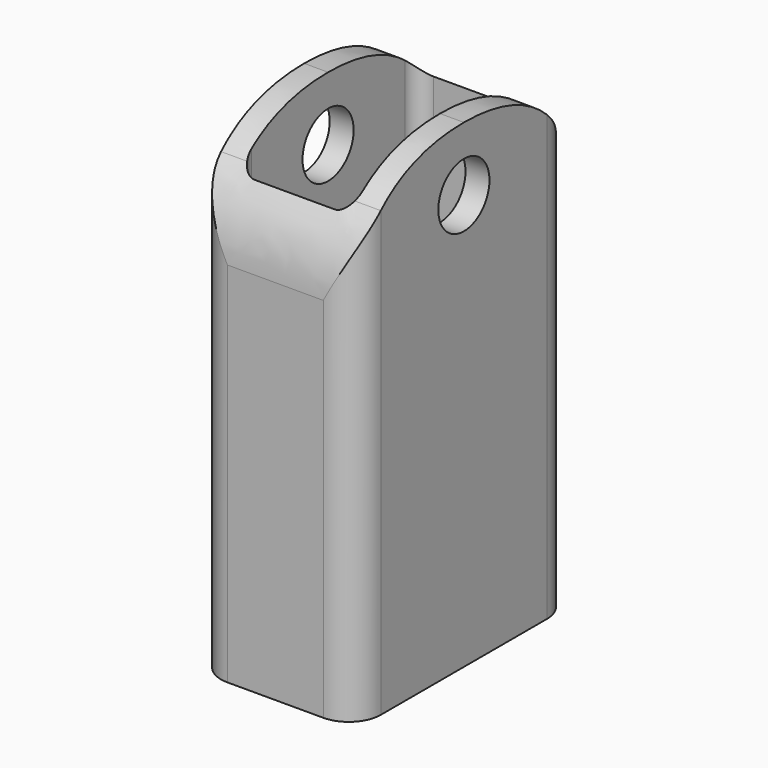
from build123d import *

# Parameters (mm, degrees)
F1_DEPTH     = 1.4
F2_DEPTH     = 30
F3_R         = 2
F4_DEPTH     = 10.001
F5_T4_DEPTH  = 22
F5_T10_DEPTH = 22


# Not quite as in the source:
# - a fillet or chamfer that OpenCascade refuses, or shapes differently, is made with other operations: its cross-section is extruded or revolved along the edge and cut away or added


with BuildPart() as f1:
    # F0 (on Top) → F1 (new body)
    with BuildSketch(Plane.XY):
        with BuildLine():
            ThreePointArc((5, 6.5), (4.4142135624, 7.9142135624), (3, 8.5))
            Line((3, 8.5), (-3, 8.5))
            ThreePointArc((-3, 8.5), (-4.4142135624, 7.9142135624), (-5, 6.5))
            Line((-5, 6.5), (-5, -6.5))
            ThreePointArc((-5, -6.5), (-4.4142135624, -7.9142135624), (-3, -8.5))
            Line((-3, -8.5), (3, -8.5))
            ThreePointArc((3, -8.5), (4.4142135624, -7.9142135624), (5, -6.5))
            Line((5, -6.5), (5, 6.5))
        make_face()
        with BuildLine():
            Line((-2.5, 7), (2.5, 7))
            ThreePointArc((2.5, 7), (3.2071067812, 6.7071067812), (3.5, 6))
            Line((3.5, 6), (3.5, -6))
            ThreePointArc((3.5, -6), (3.2071067812, -6.7071067812), (2.5, -7))
            Line((2.5, -7), (-2.5, -7))
            ThreePointArc((-2.5, -7), (-3.2071067812, -6.7071067812), (-3.5, -6))
            Line((-3.5, -6), (-3.5, 6))
            ThreePointArc((-3.5, 6), (-3.2071067812, 6.7071067812), (-2.5, 7))
        make_face(mode=Mode.SUBTRACT)
        with BuildLine():
            ThreePointArc((3.5, 6), (3.2071067812, 6.7071067812), (2.5, 7))
            Line((2.5, 7), (-2.5, 7))
            ThreePointArc((-2.5, 7), (-3.2071067812, 6.7071067812), (-3.5, 6))
            Line((-3.5, 6), (-3.5, -6))
            ThreePointArc((-3.5, -6), (-3.2071067812, -6.7071067812), (-2.5, -7))
            Line((-2.5, -7), (2.5, -7))
            ThreePointArc((2.5, -7), (3.2071067812, -6.7071067812), (3.5, -6))
            Line((3.5, -6), (3.5, 6))
        make_face()
    extrude(amount=F1_DEPTH)

    # F0 (on Top) → F2 (join)
    with BuildSketch(Plane.XY):
        with BuildLine():
            ThreePointArc((5, 6.5), (4.4142135624, 7.9142135624), (3, 8.5))
            Line((3, 8.5), (-3, 8.5))
            ThreePointArc((-3, 8.5), (-4.4142135624, 7.9142135624), (-5, 6.5))
            Line((-5, 6.5), (-5, -6.5))
            ThreePointArc((-5, -6.5), (-4.4142135624, -7.9142135624), (-3, -8.5))
            Line((-3, -8.5), (3, -8.5))
            ThreePointArc((3, -8.5), (4.4142135624, -7.9142135624), (5, -6.5))
            Line((5, -6.5), (5, 6.5))
        make_face()
        with BuildLine():
            Line((-2.5, 7), (2.5, 7))
            ThreePointArc((2.5, 7), (3.2071067812, 6.7071067812), (3.5, 6))
            Line((3.5, 6), (3.5, -6))
            ThreePointArc((3.5, -6), (3.2071067812, -6.7071067812), (2.5, -7))
            Line((2.5, -7), (-2.5, -7))
            ThreePointArc((-2.5, -7), (-3.2071067812, -6.7071067812), (-3.5, -6))
            Line((-3.5, -6), (-3.5, 6))
            ThreePointArc((-3.5, 6), (-3.2071067812, 6.7071067812), (-2.5, 7))
        make_face(mode=Mode.SUBTRACT)
    extrude(amount=F2_DEPTH)

    # F3 (on face) → F4 (cut, through all)
    with BuildSketch(Plane.YZ.offset(5)):
        with BuildLine():
            Line((-6.5, 30), (-8.5, 30))
            Line((-8.5, 30), (-8.5, 23))
            add(Edge.make_bspline(
                [(-8.5, 23), (-8.5, 24.7288344073), (-7.8671961607, 26.4695503036), (-6.5, 27.7826630238)],
                knots=[0, 0, 0, 0, 5.4766681565, 5.4766681565, 5.4766681565, 5.4766681565], degree=3))
            Line((-6.5, 27.7826630238), (-6.5, 30))
        make_face()
        with BuildLine():
            Line((0, 30), (-6.5, 30))
            Line((-6.5, 30), (-6.5, 27.7826630238))
            add(Edge.make_bspline(
                [(-6.5, 27.7826630238), (-5.1183193544, 29.1096872527), (-2.9866032163, 30), (0, 30)],
                knots=[5.4766681565, 5.4766681565, 5.4766681565, 5.4766681565, 11.0113577728, 11.0113577728, 11.0113577728, 11.0113577728], degree=3))
        make_face()
        with BuildLine():
            Line((6.5, 30), (0, 30))
            add(Edge.make_bspline(
                [(6.5, 27.7826630238), (5.1183193544, 29.1096872527), (2.9866032163, 30), (0, 30)],
                knots=[5.4766681565, 5.4766681565, 5.4766681565, 5.4766681565, 11.0113577728, 11.0113577728, 11.0113577728, 11.0113577728], degree=3))
            Line((6.5, 27.7826630238), (6.5, 30))
        make_face()
        with BuildLine():
            Line((6.5, 30), (6.5, 27.7826630238))
            add(Edge.make_bspline(
                [(8.5, 23), (8.5, 24.7288344073), (7.8671961607, 26.4695503036), (6.5, 27.7826630238)],
                knots=[0, 0, 0, 0, 5.4766681565, 5.4766681565, 5.4766681565, 5.4766681565], degree=3))
            Line((8.5, 23), (8.5, 30))
            Line((8.5, 30), (6.5, 30))
        make_face()
        with Locations((0, 26)):
            Circle(F3_R)
    extrude(amount=-F4_DEPTH, mode=Mode.SUBTRACT)

    # F5: fillet of radius 2 on 2 edges, made by hand


with BuildPart() as f5_tool2:
    # F5_s3 → F5_t4 (new body)
    with BuildSketch(Plane.XZ.offset(11)):
        with BuildLine():
            ThreePointArc((3.5, 3.4), (2.9142135624, 1.9857864376), (1.5, 1.4))
            Line((1.5, 1.4), (3.5, 1.4))
            Line((3.5, 1.4), (3.5, 3.4))
        make_face()
    extrude(amount=-F5_T4_DEPTH)

    split(bisect_by=Plane.XZ.offset(7), keep=Keep.BOTTOM)

    split(bisect_by=Plane.XZ.offset(-7), keep=Keep.TOP)


with BuildPart() as f1_1:
    add(f1.part)

    # F5_t1: union F5_tool2
    add(f5_tool2.part)


with BuildPart() as f5_tool8:
    # F5_s9 → F5_t10 (new body)
    with BuildSketch(Plane.XZ.offset(-11)):
        with BuildLine():
            ThreePointArc((-1.5, 1.4), (-2.9142135624, 1.9857864376), (-3.5, 3.4))
            Line((-3.5, 3.4), (-3.5, 1.4))
            Line((-3.5, 1.4), (-1.5, 1.4))
        make_face()
    extrude(amount=F5_T10_DEPTH)

    split(bisect_by=Plane.XZ.offset(7), keep=Keep.BOTTOM)

    split(bisect_by=Plane.XZ.offset(-7), keep=Keep.TOP)


with BuildPart() as f1_2:
    add(f1_1.part)

    # F5_t7: union F5_tool8
    add(f5_tool8.part)


solid = f1_2.part
